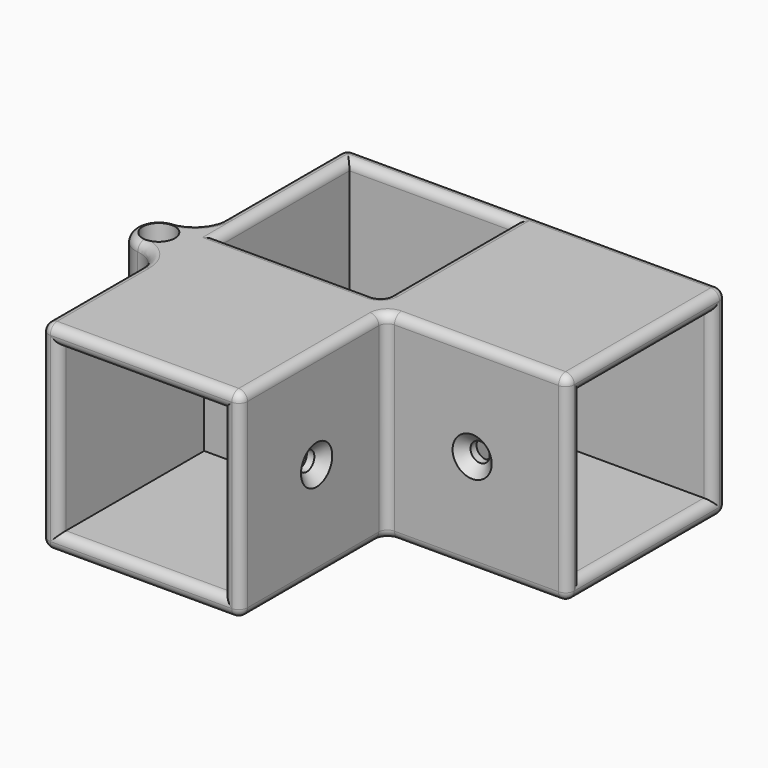
from build123d import *

# Parameters (mm, degrees)
F0_W                  = 34.2
F0_H                  = 34.2
F0_W_2                = 28.2
F0_H_2                = 28.2
F1_DEPTH              = 3
F2_DEPTH              = 31.2
F3_W                  = 34.2
F3_H                  = 34.2
F3_W_2                = 28.2
F3_H_2                = 28.2
F4_DEPTH              = 31.2
F5_W                  = 34.2
F5_H                  = 34.2
F5_W_2                = 28.2
F5_H_2                = 28.2
F6_DEPTH              = 31.2
F7_D                  = 3.3
F7_DEPTH              = 13.5
F7_CSINK_D            = 6.72
F7_CSINK_ANGLE        = 90
F7_TIP                = 0.9914200214
F7_ON_F3_D            = 3.3
F7_ON_F3_DEPTH        = 13.5
F7_ON_F3_CSINK_D      = 6.72
F7_ON_F3_CSINK_ANGLE  = 90
F7_ON_F3_TIP          = 0.9914200214
F10_D                 = 3.3
F10_DEPTH             = 13.5
F10_CSINK_D           = 6.72
F10_CSINK_ANGLE       = 90
F10_TIP               = 0.9914200214
F10_ON_F8_D           = 3.3
F10_ON_F8_DEPTH       = 13.5
F10_ON_F8_CSINK_D     = 6.72
F10_ON_F8_CSINK_ANGLE = 90
F10_ON_F8_TIP         = 0.9914200214
F12_DEPTH             = 34.2
F13_R                 = 5
F14_R                 = 1.49999
F15_D                 = 5.5


# Not quite as in the source:
# - a fillet or chamfer is up to 0.001 mm smaller than in the source, because OpenCascade refuses the exact size


with BuildPart() as f1:
    # F0 (on Top) → F1 (new body)
    with BuildSketch(Plane.XY):
        with Locations((-14.1, 14.1)):
            Rectangle(F0_W, F0_H)
        with Locations((-14.1, 14.1)):
            Rectangle(F0_W_2, F0_H_2, mode=Mode.SUBTRACT)
        with Locations((-14.1, 14.1)):
            Rectangle(F0_W_2, F0_H_2)
    extrude(amount=-F1_DEPTH)

    # F0 (on Top) → F2 (join)
    with BuildSketch(Plane.XY):
        with Locations((-14.1, 14.1)):
            Rectangle(F0_W, F0_H)
        with Locations((-14.1, 14.1)):
            Rectangle(F0_W_2, F0_H_2, mode=Mode.SUBTRACT)
    extrude(amount=F2_DEPTH)

    # F3 (on face) → F4 (join)
    with BuildSketch(Plane.XZ.offset(3)):
        with Locations((-14.1, 14.1)):
            Rectangle(F3_W, F3_H)
        with Locations((-14.1, 14.1)):
            Rectangle(F3_W_2, F3_H_2, mode=Mode.SUBTRACT)
    extrude(amount=F4_DEPTH)

    # F5 (on face) → F6 (join)
    with BuildSketch(Plane.YZ.offset(3)):
        with Locations((14.1, 14.1)):
            Rectangle(F5_W, F5_H)
        with Locations((14.1, 14.1)):
            Rectangle(F5_W_2, F5_H_2, mode=Mode.SUBTRACT)
    extrude(amount=F6_DEPTH)

    # F7
    with Locations(Plane.YZ.offset(3)):
        with Locations((14.1, 14.1)):
            CounterSinkHole(F7_D / 2, F7_CSINK_D / 2, depth=F7_DEPTH, counter_sink_angle=F7_CSINK_ANGLE)
            with Locations((0, 0, -(F7_DEPTH + F7_TIP / 2))):  # 118° drill point
                Cone(0, F7_D / 2, F7_TIP, mode=Mode.SUBTRACT)

    # F7 on F3
    with Locations(Plane.XZ.offset(3)):
        with Locations((-14.1, 14.1)):
            CounterSinkHole(F7_ON_F3_D / 2, F7_ON_F3_CSINK_D / 2, depth=F7_ON_F3_DEPTH, counter_sink_angle=F7_ON_F3_CSINK_ANGLE)
            with Locations((0, 0, -(F7_ON_F3_DEPTH + F7_ON_F3_TIP / 2))):  # 118° drill point
                Cone(0, F7_ON_F3_D / 2, F7_ON_F3_TIP, mode=Mode.SUBTRACT)

    # F10
    with Locations(Plane.XZ.offset(3)):
        with Locations((17.85, 14.1)):
            CounterSinkHole(F10_D / 2, F10_CSINK_D / 2, depth=F10_DEPTH, counter_sink_angle=F10_CSINK_ANGLE)
            with Locations((0, 0, -(F10_DEPTH + F10_TIP / 2))):  # 118° drill point
                Cone(0, F10_D / 2, F10_TIP, mode=Mode.SUBTRACT)

    # F10 on F8
    with Locations(Plane.YZ.offset(3)):
        with Locations((-17.85, 14.1)):
            CounterSinkHole(F10_ON_F8_D / 2, F10_ON_F8_CSINK_D / 2, depth=F10_ON_F8_DEPTH, counter_sink_angle=F10_ON_F8_CSINK_ANGLE)
            with Locations((0, 0, -(F10_ON_F8_DEPTH + F10_ON_F8_TIP / 2))):  # 118° drill point
                Cone(0, F10_ON_F8_D / 2, F10_ON_F8_TIP, mode=Mode.SUBTRACT)

    # F11 (on face) → F12 (join, through all)
    with BuildSketch(Plane.XY.offset(31.2)):
        with BuildLine():
            Line((-31.2, 0), (-35.2, 0))
            ThreePointArc((-35.2, 0), (-39.2, -4), (-35.2, -8))
            Line((-35.2, -8), (-31.2, -8))
            Line((-31.2, -8), (-31.2, 0))
        make_face()
    extrude(amount=-F12_DEPTH)

    # F13
    f13_edges = [f1.edges().sort_by_distance(p)[0] for p in [
        (-31.2, 0, 14.1),
        (-31.2, -8, 14.1),
    ]]
    fillet(f13_edges, radius=F13_R)

    # F14 (radius 1.5 in the source; OpenCascade refuses exactly that, so slightly less here)
    f14_edges = [f1.edges().sort_by_distance(p)[0] for p in [
        (-32.47322, -9.610939, -3),
        (-32.47322, -9.610939, 31.2),
        (1.5, 31.2, -3),
        (34.2, 31.2, 14.1),
        (1.5, 31.2, 31.2),
        (-31.2, 31.2, 14.1),
        (-31.2, -34.2, 14.1),
        (-14.1, -34.2, -3),
        (3, -34.2, 14.1),
        (-14.1, -34.2, 31.2),
        (-14.1, -34.2, 28.2),
        (0, -34.2, 14.1),
        (-14.1, -34.2, 0),
        (-28.2, -34.2, 14.1),
        (3, -18.6, -3),
        (3, -3, 14.1),
        (18.6, -3, -3),
        (3, -18.6, 31.2),
        (18.6, -3, 31.2),
        (34.2, -3, 14.1),
        (34.2, 14.1, -3),
        (34.2, 28.2, 14.1),
        (34.2, 14.1, 28.2),
        (34.2, 14.1, 31.2),
        (34.2, 14.1, 0),
        (34.2, 0, 14.1),
        (-14.1, 0, 31.2),
        (-28.2, 14.1, 31.2),
        (-14.1, 28.2, 31.2),
        (0, 0, 15.6),
        (-31.2, 18.072136, 31.2),
        (-31.2, 18.072136, -3),
        (-31.2, -23.572136, 31.2),
        (-39.2, -4, 31.2),
        (-32.47322, 1.610939, 31.2),
        (0, 14.1, 31.2),
        (-32.47322, 1.610939, -3),
        (-39.2, -4, -3),
        (-31.2, -23.572136, -3),
    ]]
    fillet(f14_edges, radius=F14_R)

    # F15 (through all)
    with Locations(Plane.XY.offset(31.2)):
        with Locations((-35.2, -4)):
            Hole(F15_D / 2)


solid = f1.part
